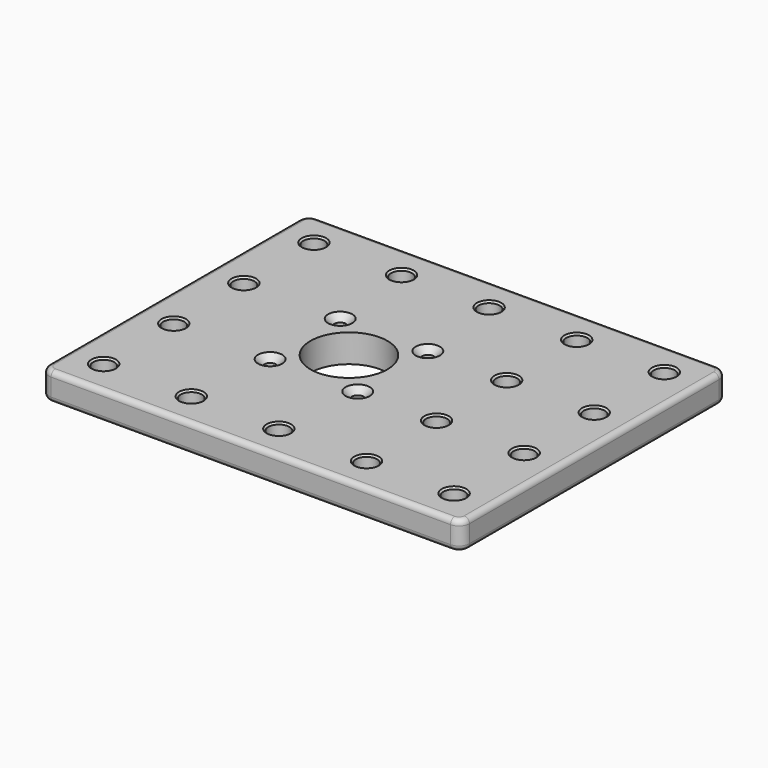
from build123d import *

# Parameters (mm, degrees)
F0_W         = 120
F0_H         = 95
F0_R         = 3
F0_R_2       = 1.65
F0_R_3       = 11
F1_DEPTH     = 8
F2_R         = 1.5
F3_SIZE      = 1.8
F4_T1_DEPTH  = 8
F4_T4_ANGLE  = 90
F4_T6_ANGLE  = 90
F4_T8_ANGLE  = 90
F4_T10_ANGLE = 90
F4_T12_ANGLE = 90
F4_T14_ANGLE = 90
F4_T16_ANGLE = 90
F4_T18_ANGLE = 90
F5_SIZE      = 0.5


# Not quite as in the source:
# - a fillet or chamfer that OpenCascade refuses, or shapes differently, is made with other operations: its cross-section is extruded or revolved along the edge and cut away or added


with BuildPart() as f1:
    # F0 (on Top) → F1 (new body)
    with BuildSketch(Plane.XY):
        with Locations((-21.1694301665, -8.1955979578)):
            Rectangle(F0_W, F0_H)
        with Locations((-71.1694301665, -45.6955979578)):
            Circle(F0_R, mode=Mode.SUBTRACT)
        with Locations((-46.1694301665, -45.6955979578)):
            Circle(F0_R, mode=Mode.SUBTRACT)
        with Locations((-21.1694301665, -45.6955979578)):
            Circle(F0_R, mode=Mode.SUBTRACT)
        with Locations((-71.1694301665, -20.6955979578)):
            Circle(F0_R, mode=Mode.SUBTRACT)
        with Locations((-43.6694301665, -20.6955979578)):
            Circle(F0_R_2, mode=Mode.SUBTRACT)
        with Locations((3.8305698335, -45.6955979578)):
            Circle(F0_R, mode=Mode.SUBTRACT)
        with Locations((28.8305698335, -45.6955979578)):
            Circle(F0_R, mode=Mode.SUBTRACT)
        with Locations((-18.6694301665, -20.6955979578)):
            Circle(F0_R_2, mode=Mode.SUBTRACT)
        with Locations((3.8305698335, -20.6955979578)):
            Circle(F0_R, mode=Mode.SUBTRACT)
        with Locations((28.8305698335, -20.6955979578)):
            Circle(F0_R, mode=Mode.SUBTRACT)
        with Locations((-71.1694301665, 4.3044020422)):
            Circle(F0_R, mode=Mode.SUBTRACT)
        with Locations((-31.1694301665, -8.1955979578)):
            Circle(F0_R_3, mode=Mode.SUBTRACT)
        with Locations((-43.6694301665, 4.3044020422)):
            Circle(F0_R_2, mode=Mode.SUBTRACT)
        with Locations((-71.1694301665, 29.3044020422)):
            Circle(F0_R, mode=Mode.SUBTRACT)
        with Locations((-46.1694301665, 29.3044020422)):
            Circle(F0_R, mode=Mode.SUBTRACT)
        with Locations((-21.1694301665, 29.3044020422)):
            Circle(F0_R, mode=Mode.SUBTRACT)
        with Locations((-18.6694301665, 4.3044020422)):
            Circle(F0_R_2, mode=Mode.SUBTRACT)
        with Locations((3.8305698335, 4.3044020422)):
            Circle(F0_R, mode=Mode.SUBTRACT)
        with Locations((28.8305698335, 4.3044020422)):
            Circle(F0_R, mode=Mode.SUBTRACT)
        with Locations((3.8305698335, 29.3044020422)):
            Circle(F0_R, mode=Mode.SUBTRACT)
        with Locations((28.8305698335, 29.3044020422)):
            Circle(F0_R, mode=Mode.SUBTRACT)
    extrude(amount=-F1_DEPTH)

    # F2
    f2_edges = [f1.edges().sort_by_distance(p)[0] for p in [
        (-21.16943, -55.695598, 0),
        (38.83057, -8.195598, 0),
        (-21.16943, 39.304402, 0),
        (-81.16943, -8.195598, 0),
        (-21.16943, -55.695598, -8),
        (38.83057, -8.195598, -8),
        (-81.16943, -8.195598, -8),
        (-21.16943, 39.304402, -8),
    ]]
    fillet(f2_edges, radius=F2_R)

    # F3
    f3_edges = [f1.edges().sort_by_distance(p)[0] for p in [
        (-45.31943, 4.304402, 0),
        (-20.31943, 4.304402, 0),
        (-20.31943, -20.695598, 0),
        (-45.31943, -20.695598, 0),
        (-45.31943, -20.695598, -8),
        (-20.31943, 4.304402, -8),
        (-20.31943, -20.695598, -8),
        (-45.31943, 4.304402, -8),
    ]]
    chamfer(f3_edges, length=F3_SIZE)

    # F4: fillet of radius 3 on 4 edges, made by hand

    # F4_s2 → F4_t1 (cut)
    with BuildSketch(Plane.XY.offset(-8)):
        with BuildLine():
            ThreePointArc((-78.1694301665, -55.6955979578), (-80.29075051, -54.8169183014), (-81.1694301665, -52.6955979578))
            Line((-81.1694301665, -52.6955979578), (-81.1694301665, -55.6955979578))
            Line((-81.1694301665, -55.6955979578), (-78.1694301665, -55.6955979578))
        make_face()
        with BuildLine():
            ThreePointArc((35.8305698335, -55.6955979578), (37.9518901771, -54.8169183014), (38.8305698335, -52.6955979578))
            Line((38.8305698335, -52.6955979578), (38.8305698335, -55.6955979578))
            Line((38.8305698335, -55.6955979578), (35.8305698335, -55.6955979578))
        make_face()
        with BuildLine():
            ThreePointArc((-81.1694301665, 36.3044020422), (-80.29075051, 38.4257223857), (-78.1694301665, 39.3044020422))
            Line((-78.1694301665, 39.3044020422), (-81.1694301665, 39.3044020422))
            Line((-81.1694301665, 39.3044020422), (-81.1694301665, 36.3044020422))
        make_face()
        with BuildLine():
            ThreePointArc((38.8305698335, 36.3044020422), (37.9518901771, 38.4257223857), (35.8305698335, 39.3044020422))
            Line((35.8305698335, 39.3044020422), (38.8305698335, 39.3044020422))
            Line((38.8305698335, 39.3044020422), (38.8305698335, 36.3044020422))
        make_face()
    extrude(amount=F4_T1_DEPTH, mode=Mode.SUBTRACT)

    # F4_s3 → F4_t4 (revolve, cut)
    with BuildSketch(Plane.XZ.offset(-36.3044020422)):
        with BuildLine():
            ThreePointArc((37.3305698335, 0), (38.3912300053, -0.4393398282), (38.8305698335, -1.5))
            Line((38.8305698335, -1.5), (38.8305698335, 0))
            Line((38.8305698335, 0), (37.3305698335, 0))
        make_face()
    revolve(axis=Axis((35.8305698335, 36.3044020422, 0), (0, 0, 1)), revolution_arc=F4_T4_ANGLE, mode=Mode.SUBTRACT)

    # F4_s5 → F4_t6 (revolve, cut)
    with BuildSketch(Plane.YZ.offset(35.8305698335)):
        with BuildLine():
            ThreePointArc((37.8044020422, -8), (38.865062214, -7.5606601718), (39.3044020422, -6.5))
            Line((39.3044020422, -6.5), (39.3044020422, -8))
            Line((39.3044020422, -8), (37.8044020422, -8))
        make_face()
    revolve(axis=Axis((35.8305698335, 36.3044020422, -8), (0, 0, -1)), revolution_arc=F4_T6_ANGLE, mode=Mode.SUBTRACT)

    # F4_s7 → F4_t8 (revolve, cut)
    with BuildSketch(Plane.YZ.offset(-78.1694301665)):
        with BuildLine():
            ThreePointArc((37.8044020422, 0), (38.865062214, -0.4393398282), (39.3044020422, -1.5))
            Line((39.3044020422, -1.5), (39.3044020422, 0))
            Line((39.3044020422, 0), (37.8044020422, 0))
        make_face()
    revolve(axis=Axis((-78.1694301665, 36.3044020422, 0), (0, 0, 1)), revolution_arc=F4_T8_ANGLE, mode=Mode.SUBTRACT)

    # F4_s9 → F4_t10 (revolve, cut)
    with BuildSketch(Plane.XZ.offset(-36.3044020422)):
        with BuildLine():
            ThreePointArc((-79.6694301665, -8), (-80.7300903383, -7.5606601718), (-81.1694301665, -6.5))
            Line((-81.1694301665, -6.5), (-81.1694301665, -8))
            Line((-81.1694301665, -8), (-79.6694301665, -8))
        make_face()
    revolve(axis=Axis((-78.1694301665, 36.3044020422, -8), (0, 0, -1)), revolution_arc=F4_T10_ANGLE, mode=Mode.SUBTRACT)

    # F4_s11 → F4_t12 (revolve, cut)
    with BuildSketch(Plane.YZ.offset(35.8305698335)):
        with BuildLine():
            ThreePointArc((-54.1955979578, 0), (-55.2562581296, -0.4393398282), (-55.6955979578, -1.5))
            Line((-55.6955979578, -1.5), (-55.6955979578, 0))
            Line((-55.6955979578, 0), (-54.1955979578, 0))
        make_face()
    revolve(axis=Axis((35.8305698335, -52.6955979578, 0), (0, 0, 1)), revolution_arc=F4_T12_ANGLE, mode=Mode.SUBTRACT)

    # F4_s13 → F4_t14 (revolve, cut)
    with BuildSketch(Plane.XZ.offset(52.6955979578)):
        with BuildLine():
            ThreePointArc((37.3305698335, -8), (38.3912300053, -7.5606601718), (38.8305698335, -6.5))
            Line((38.8305698335, -6.5), (38.8305698335, -8))
            Line((38.8305698335, -8), (37.3305698335, -8))
        make_face()
    revolve(axis=Axis((35.8305698335, -52.6955979578, -8), (0, 0, -1)), revolution_arc=F4_T14_ANGLE, mode=Mode.SUBTRACT)

    # F4_s15 → F4_t16 (revolve, cut)
    with BuildSketch(Plane.XZ.offset(52.6955979578)):
        with BuildLine():
            ThreePointArc((-79.6694301665, 0), (-80.7300903383, -0.4393398282), (-81.1694301665, -1.5))
            Line((-81.1694301665, -1.5), (-81.1694301665, 0))
            Line((-81.1694301665, 0), (-79.6694301665, 0))
        make_face()
    revolve(axis=Axis((-78.1694301665, -52.6955979578, 0), (0, 0, 1)), revolution_arc=F4_T16_ANGLE, mode=Mode.SUBTRACT)

    # F4_s17 → F4_t18 (revolve, cut)
    with BuildSketch(Plane.YZ.offset(-78.1694301665)):
        with BuildLine():
            ThreePointArc((-54.1955979578, -8), (-55.2562581296, -7.5606601718), (-55.6955979578, -6.5))
            Line((-55.6955979578, -6.5), (-55.6955979578, -8))
            Line((-55.6955979578, -8), (-54.1955979578, -8))
        make_face()
    revolve(axis=Axis((-78.1694301665, -52.6955979578, -8), (0, 0, -1)), revolution_arc=F4_T18_ANGLE, mode=Mode.SUBTRACT)

    # F5
    f5_edges = [f1.edges().sort_by_distance(p)[0] for p in [
        (-74.16943, -45.695598, -8),
        (-74.16943, -45.695598, 0),
        (25.83057, -45.695598, -8),
        (0.83057, -45.695598, -8),
        (-49.16943, -45.695598, -8),
        (-24.16943, -45.695598, -8),
        (0.83057, -45.695598, 0),
        (25.83057, -45.695598, 0),
        (-24.16943, -45.695598, 0),
        (-49.16943, -45.695598, 0),
        (25.83057, 4.304402, -8),
        (0.83057, 4.304402, -8),
        (0.83057, -20.695598, -8),
        (0.83057, 4.304402, 0),
        (25.83057, -20.695598, -8),
        (25.83057, 29.304402, -8),
        (0.83057, -20.695598, 0),
        (0.83057, 29.304402, -8),
        (25.83057, 4.304402, 0),
        (0.83057, 29.304402, 0),
        (25.83057, 29.304402, 0),
        (25.83057, -20.695598, 0),
        (-24.16943, 29.304402, -8),
        (-49.16943, 29.304402, -8),
        (-74.16943, 29.304402, -8),
        (-24.16943, 29.304402, 0),
        (-49.16943, 29.304402, 0),
        (-74.16943, 29.304402, 0),
        (-74.16943, 4.304402, -8),
        (-74.16943, -20.695598, -8),
        (-74.16943, -20.695598, 0),
        (-74.16943, 4.304402, 0),
    ]]
    chamfer(f5_edges, length=F5_SIZE)


solid = f1.part
